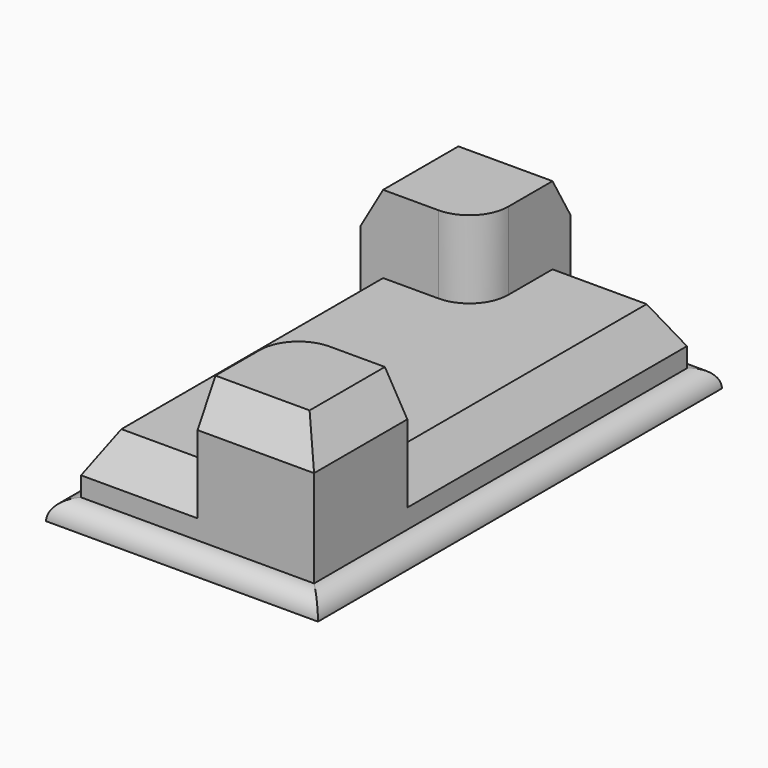
from build123d import *

# Parameters (mm, degrees)
F0_W     = 88.8999994576
F0_H     = 165.0999994576
F1_DEPTH = 6.35
F2_DEPTH = 25.4
F3_DEPTH = 50.8
F4_R     = 6.34999
F5_SIZE2 = 12.7
F5_SIZE  = 7.3323484187
F6_SIZE2 = 12.7
F6_SIZE  = 7.3323484187
F7_SIZE2 = 12.7
F7_SIZE  = 7.3323484187
F8_SIZE2 = 12.7
F8_SIZE  = 7.3323484187


# Not quite as in the source:
# - a fillet or chamfer is up to 0.001 mm smaller than in the source, because OpenCascade refuses the exact size


with BuildPart() as f1:
    # F0 (on Top) → F1 (new body)
    with BuildSketch(Plane.XY):
        with Locations((-2.712e-07, -2.712e-07)):
            Rectangle(F0_W, F0_H)
        Polygon((38.1, -38.1), (38.1, -76.2), (0, -76.2), (-38.1, -76.2), (-38.1, 38.1), (-38.1, 76.2), (0, 76.2), (38.1, 76.2), align=None, mode=Mode.SUBTRACT)
        with BuildLine():
            Line((-38.1, -76.2), (0, -76.2))
            Line((0, -76.2), (0, -50.8))
            ThreePointArc((0, -50.8), (3.7197438789, -41.8197438789), (12.7, -38.1))
            Line((12.7, -38.1), (38.1, -38.1))
            Line((38.1, -38.1), (38.1, 76.2))
            Line((38.1, 76.2), (0, 76.2))
            Line((0, 76.2), (0, 50.8))
            ThreePointArc((0, 50.8), (-3.7197438789, 41.8197438789), (-12.7, 38.1))
            Line((-12.7, 38.1), (-38.1, 38.1))
            Line((-38.1, 38.1), (-38.1, -76.2))
        make_face()
        with BuildLine():
            Line((0, -76.2), (38.1, -76.2))
            Line((38.1, -76.2), (38.1, -38.1))
            Line((38.1, -38.1), (12.7, -38.1))
            ThreePointArc((12.7, -38.1), (3.7197438789, -41.8197438789), (0, -50.8))
            Line((0, -50.8), (0, -76.2))
        make_face()
        with BuildLine():
            Line((-38.1, 76.2), (-38.1, 38.1))
            Line((-38.1, 38.1), (-12.7, 38.1))
            ThreePointArc((-12.7, 38.1), (-3.7197438789, 41.8197438789), (0, 50.8))
            Line((0, 50.8), (0, 76.2))
            Line((0, 76.2), (-38.1, 76.2))
        make_face()
    extrude(amount=F1_DEPTH)

    # F0 (on Top) → F2 (join)
    with BuildSketch(Plane.XY):
        with BuildLine():
            Line((-38.1, 76.2), (-38.1, 38.1))
            Line((-38.1, 38.1), (-12.7, 38.1))
            ThreePointArc((-12.7, 38.1), (-3.7197438789, 41.8197438789), (0, 50.8))
            Line((0, 50.8), (0, 76.2))
            Line((0, 76.2), (-38.1, 76.2))
        make_face()
        with BuildLine():
            Line((-38.1, -76.2), (0, -76.2))
            Line((0, -76.2), (0, -50.8))
            ThreePointArc((0, -50.8), (3.7197438789, -41.8197438789), (12.7, -38.1))
            Line((12.7, -38.1), (38.1, -38.1))
            Line((38.1, -38.1), (38.1, 76.2))
            Line((38.1, 76.2), (0, 76.2))
            Line((0, 76.2), (0, 50.8))
            ThreePointArc((0, 50.8), (-3.7197438789, 41.8197438789), (-12.7, 38.1))
            Line((-12.7, 38.1), (-38.1, 38.1))
            Line((-38.1, 38.1), (-38.1, -76.2))
        make_face()
        with BuildLine():
            Line((0, -76.2), (38.1, -76.2))
            Line((38.1, -76.2), (38.1, -38.1))
            Line((38.1, -38.1), (12.7, -38.1))
            ThreePointArc((12.7, -38.1), (3.7197438789, -41.8197438789), (0, -50.8))
            Line((0, -50.8), (0, -76.2))
        make_face()
    extrude(amount=F2_DEPTH)

    # F0 (on Top) → F3 (join)
    with BuildSketch(Plane.XY):
        with BuildLine():
            Line((0, -76.2), (38.1, -76.2))
            Line((38.1, -76.2), (38.1, -38.1))
            Line((38.1, -38.1), (12.7, -38.1))
            ThreePointArc((12.7, -38.1), (3.7197438789, -41.8197438789), (0, -50.8))
            Line((0, -50.8), (0, -76.2))
        make_face()
        with BuildLine():
            Line((-38.1, 76.2), (-38.1, 38.1))
            Line((-38.1, 38.1), (-12.7, 38.1))
            ThreePointArc((-12.7, 38.1), (-3.7197438789, 41.8197438789), (0, 50.8))
            Line((0, 50.8), (0, 76.2))
            Line((0, 76.2), (-38.1, 76.2))
        make_face()
    extrude(amount=F3_DEPTH)

    # F4 (radius 6.35 in the source; OpenCascade refuses exactly that, so slightly less here)
    f4_edges = [f1.edges().sort_by_distance(p)[0] for p in [
        (-44.45, 0, 6.35),
        (0, -82.55, 6.35),
        (44.449999, 0, 6.35),
        (0, 82.549999, 6.35),
    ]]
    fillet(f4_edges, radius=F4_R)

    # F5
    f5_edges = [f1.edges().sort_by_distance(p)[0] for p in [
        (-38.1, 57.15, 50.8),
        (-19.05, 76.2, 50.8),
    ]]
    f5_side = f1.faces().sort_by_distance((-19.446042, 57.546042, 50.8))[0]
    chamfer(f5_edges, length=F5_SIZE, length2=F5_SIZE2, reference=f5_side)

    # F6
    f6_edges = [f1.edges().sort_by_distance(p)[0] for p in [
        (19.05, -76.2, 50.8),
        (38.1, -57.15, 50.8),
    ]]
    f6_side = f1.faces().sort_by_distance((19.446042, -57.546042, 50.8))[0]
    chamfer(f6_edges, length=F6_SIZE, length2=F6_SIZE2, reference=f6_side)

    # F7
    f7_edges = [f1.edges().sort_by_distance(p)[0] for p in [
        (-19.05, -76.2, 25.4),
        (-38.1, -19.05, 25.4),
    ]]
    f7_side = f1.faces().sort_by_distance((0, 0, 25.4))[0]
    chamfer(f7_edges, length=F7_SIZE, length2=F7_SIZE2, reference=f7_side)

    # F8
    f8_edges = [f1.edges().sort_by_distance(p)[0] for p in [
        (38.1, 19.05, 25.4),
        (19.05, 76.2, 25.4),
    ]]
    f8_side = f1.faces().sort_by_distance((4.190317, 4.190317, 25.4))[0]
    chamfer(f8_edges, length=F8_SIZE, length2=F8_SIZE2, reference=f8_side)


solid = f1.part
